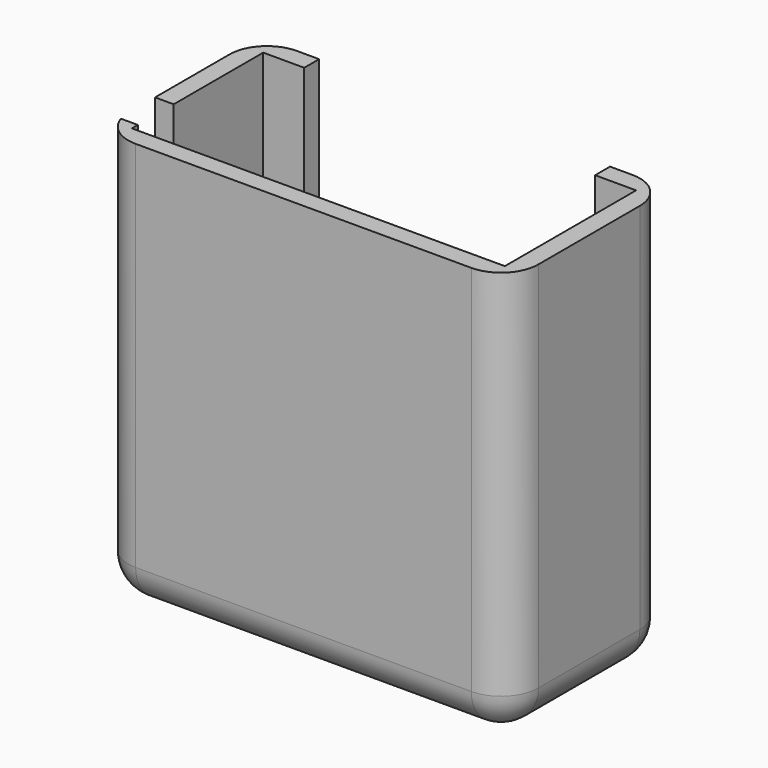
from build123d import *

# Parameters (mm, degrees)
F0_W     = 39
F0_H     = 7.6218599584
F0_H_2   = 2.5
F0_W_2   = 6.4553316683
F0_H_3   = 6
F0_W_3   = 2.5
F1_DEPTH = 5
F2_DEPTH = 55
F3_R     = 4.99999


# Not quite as in the source:
# - a fillet or chamfer is up to 0.001 mm smaller than in the source, because OpenCascade refuses the exact size


with BuildPart() as f1:
    # F0 (on Top) → F1 (new body)
    with BuildSketch(Plane.XY):
        Polygon((27.5, 13.5), (19.5, 13.5), (19.5, 11), (25, 11), (25, -11), (-25, -11), (-25, -10), (-27.5, -10), (-27.5, -13.5), (27.5, -13.5), align=None)
        Polygon((-19.5, 13.5), (-27.5, 13.5), (-27.5, -4), (-25, -4), (-25, 11), (-19.5, 11), align=None)
        Polygon((-19.5, 3.3781400416), (-19.5, 11), (-25, 11), (-25, -4), (-18.5446683317, -4), (-18.5446683317, -10), (-25, -10), (-25, -11), (25, -11), (25, 11), (19.5, 11), (19.5, 3.3781400416), align=None)
        with Locations((0, 7.1890700208)):
            Rectangle(F0_W, F0_H)
        with Locations((0, 12.25)):
            Rectangle(F0_W, F0_H_2)
        with Locations((-21.7723341659, -7)):
            Rectangle(F0_W_2, F0_H_3)
        with Locations((-26.25, -7)):
            Rectangle(F0_W_3, F0_H_3)
    extrude(amount=F1_DEPTH)

    # F0 (on Top) → F2 (join)
    with BuildSketch(Plane.XY):
        Polygon((27.5, 13.5), (19.5, 13.5), (19.5, 11), (25, 11), (25, -11), (-25, -11), (-25, -10), (-27.5, -10), (-27.5, -13.5), (27.5, -13.5), align=None)
        Polygon((-19.5, 13.5), (-27.5, 13.5), (-27.5, -4), (-25, -4), (-25, 11), (-19.5, 11), align=None)
    extrude(amount=F2_DEPTH)

    # F3 (radius 5 in the source; OpenCascade refuses exactly that, so slightly less here)
    f3_edges = [f1.edges().sort_by_distance(p)[0] for p in [
        (27.5, 13.5, 27.5),
        (-27.5, 13.5, 27.5),
        (-27.5, -13.5, 27.5),
        (27.5, -13.5, 27.5),
        (-27.5, 0, 0),
        (0, 13.5, 0),
        (27.5, 0, 0),
        (0, -13.5, 0),
    ]]
    fillet(f3_edges, radius=F3_R)


solid = f1.part
